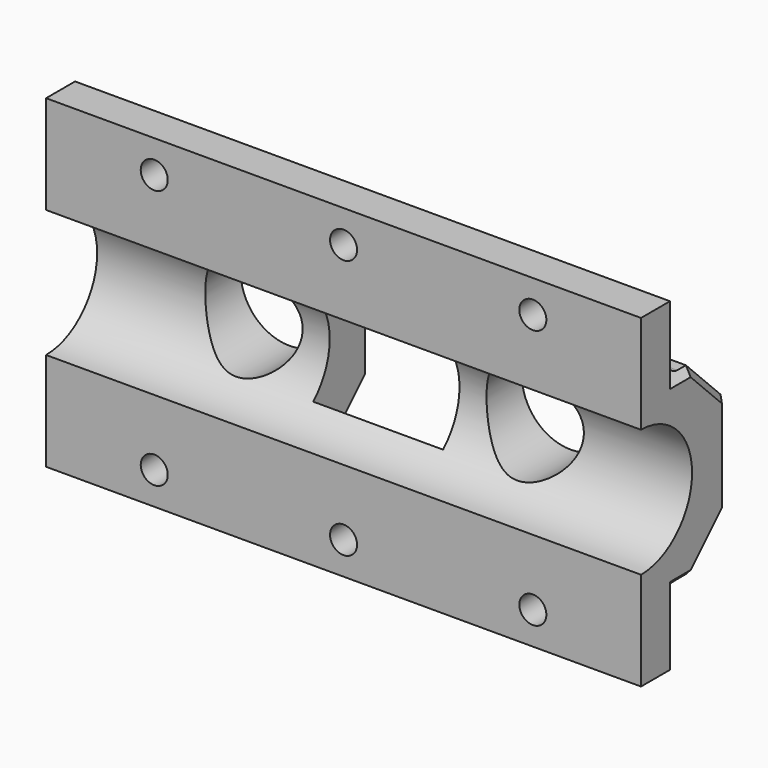
from build123d import *

# Parameters (mm, degrees)
F0_W      = 34.925
F0_H      = 12.7
F1_DEPTH  = 10.795
F2_DEPTH  = 10.795
F3_W      = 34.925
F3_H      = 19.05
F4_DEPTH  = 5.08
F5_R      = 7.493
F6_DEPTH  = 101.6
F7_R      = 1.5875
F8_DEPTH  = 25.4
F9_SIZE   = 5.08
F10_SIZE  = 0.8255
F11_R     = 1.27
F12_R     = 5.715
F13_DEPTH = 25.4
F14_W     = 7.62
F14_H     = 5.08
F15_DEPTH = 7.62


with BuildPart() as f1:
    # F0 (on Top) → F1 (new body)
    with BuildSketch(Plane.XY):
        with Locations((-17.4625, 6.35)):
            Rectangle(F0_W, F0_H)
        with Locations((17.4625, 6.35)):
            Rectangle(F0_W, F0_H)
    extrude(amount=F1_DEPTH)

    # F0 (on Top) → F2 (join)
    with BuildSketch(Plane.XY):
        with Locations((-17.4625, 6.35)):
            Rectangle(F0_W, F0_H)
        with Locations((17.4625, 6.35)):
            Rectangle(F0_W, F0_H)
    extrude(amount=-F2_DEPTH)

    # F3 (on Front) → F4 (join)
    with BuildSketch(Plane.XZ):
        with Locations((-17.4625, 9.525)):
            Rectangle(F3_W, F3_H)
        with Locations((-17.4625, -9.525)):
            Rectangle(F3_W, F3_H)
        Polygon((0, 19.05), (0, 0), (0, -19.05), (34.925, -19.05), (34.925, 0), (34.925, 19.05), align=None)
    extrude(amount=-F4_DEPTH)

    # F5 (on face) → F6 (cut)
    with BuildSketch(Plane.YZ.offset(34.925)):
        Circle(F5_R)
    extrude(amount=-F6_DEPTH, mode=Mode.SUBTRACT)

    # F7 (on face) → F8 (cut)
    with BuildSketch(Plane(origin=(0, 12.7, 0), x_dir=(-1, 0, 0), z_dir=(0, 1, 0))):
        with Locations((-22.225, -15.24)):
            Circle(F7_R)
        with Locations((-22.225, 15.24)):
            Circle(F7_R)
        with Locations((0, -15.24)):
            Circle(F7_R)
        with Locations((22.225, 15.24)):
            Circle(F7_R)
        with Locations((22.225, -15.24)):
            Circle(F7_R)
        with Locations((0, 15.24)):
            Circle(F7_R)
    extrude(amount=-F8_DEPTH, mode=Mode.SUBTRACT)

    # F9
    f9_edges = [f1.edges().sort_by_distance(p)[0] for p in [
        (0, 12.7, -10.795),
        (0, 12.7, 10.795),
    ]]
    chamfer(f9_edges, length=F9_SIZE)

    # F10
    f10_edges = [f1.edges().sort_by_distance(p)[0] for p in [
        (0, 5.08, -19.05),
        (-34.925, 5.08, -14.9225),
        (-34.925, 10.16, 8.255),
        (-34.925, 12.7, 0),
        (-34.925, 10.16, -8.255),
        (34.925, 10.16, 8.255),
        (34.925, 12.7, 0),
        (34.925, 10.16, -8.255),
        (34.925, 6.35, -10.795),
        (34.925, 5.08, -14.9225),
        (0, 5.08, 19.05),
        (-34.925, 5.08, 14.9225),
        (-34.925, 6.35, 10.795),
        (34.925, 5.08, 14.9225),
        (34.925, 6.35, 10.795),
        (-34.925, 6.35, -10.795),
    ]]
    chamfer(f10_edges, length=F10_SIZE)

    # F11
    f11_edges = [f1.edges().sort_by_distance(p)[0] for p in [
        (0, 5.08, -10.795),
        (0, 5.08, 10.795),
    ]]
    fillet(f11_edges, radius=F11_R)

    # F12 (on face) → F13 (cut)
    with BuildSketch(Plane(origin=(0, 12.7, 0), x_dir=(-1, 0, 0), z_dir=(0, 1, 0))):
        with Locations((-16.51, 0)):
            Circle(F12_R)
        with Locations((16.51, 0)):
            Circle(F12_R)
    extrude(amount=-F13_DEPTH, mode=Mode.SUBTRACT)

    # F14 (on face) → F15 (cut)
    with BuildSketch(Plane(origin=(0, 12.7, 0), x_dir=(-1, 0, 0), z_dir=(0, 1, 0))):
        Polygon((0, -5.715), (0, 0), (0, 5.715), (-7.62, 5.715), (-7.62, -5.715), align=None)
        Polygon((0, 5.715), (0, 0), (0, -5.715), (7.62, -5.715), (7.62, 5.715), align=None)
        with Locations((3.81, 8.255)):
            Rectangle(F14_W, F14_H)
        with Locations((-3.81, 8.255)):
            Rectangle(F14_W, F14_H)
        with Locations((-3.81, -8.255)):
            Rectangle(F14_W, F14_H)
        with Locations((3.81, -8.255)):
            Rectangle(F14_W, F14_H)
    extrude(amount=-F15_DEPTH, mode=Mode.SUBTRACT)


solid = f1.part
